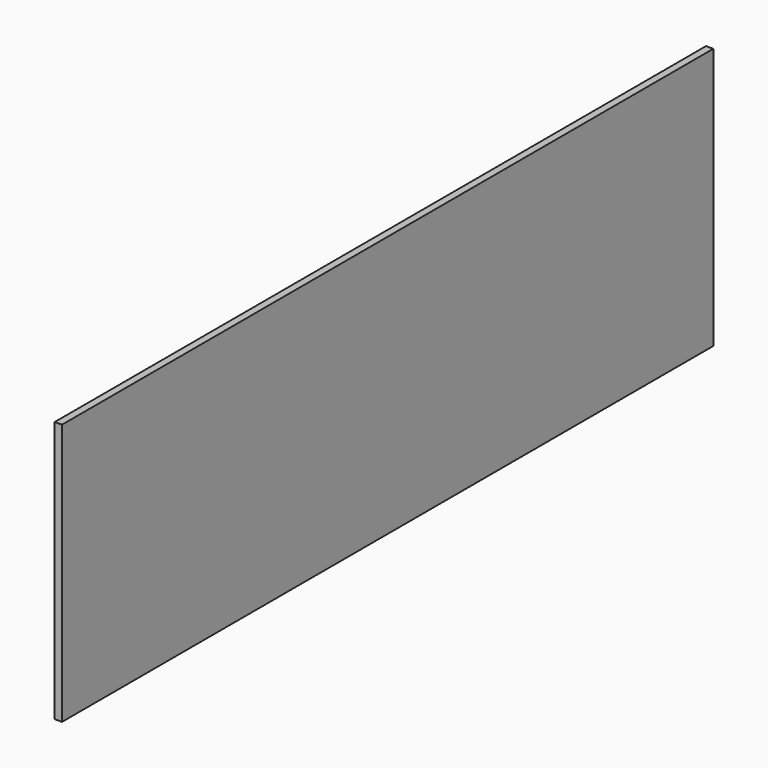
from build123d import *

# Parameters (mm, degrees)
F0_W     = 533.4
F0_H     = 171.45
F1_DEPTH = 4.7625


# Not quite as in the source:
# - a length typed as a fraction of an inch, garbled in the dataset ("3 / 203.2 mm" for 3/8 in), is restored


with BuildPart() as f1:
    # F0 (on Right) → F1 (new body)
    with BuildSketch(Plane.YZ):
        with Locations((-60.8702084428, 18.5321049437)):
            Rectangle(F0_W, F0_H)
    extrude(amount=-F1_DEPTH)


solid = f1.part
